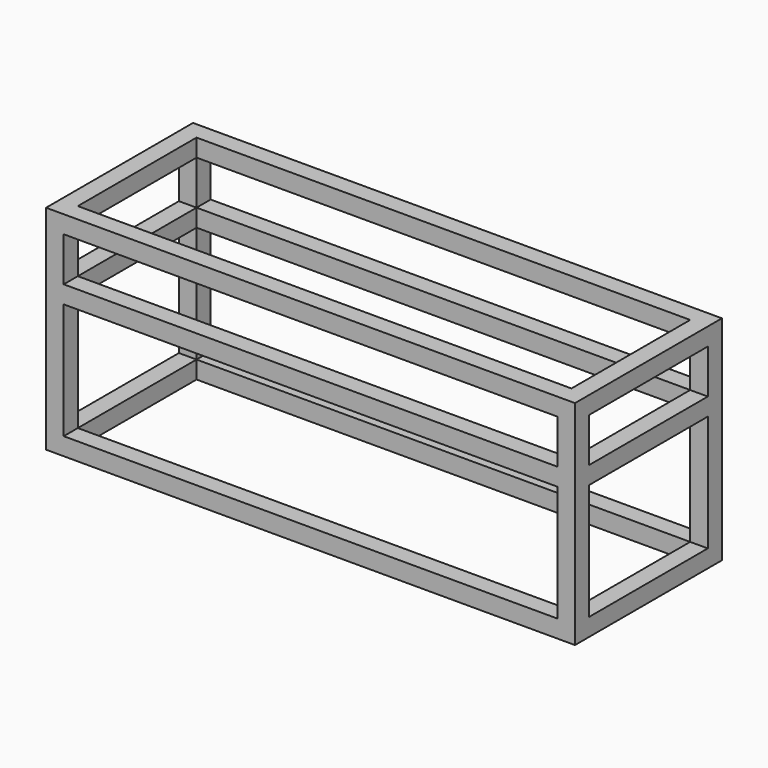
from build123d import *

# Parameters (mm, degrees)
F0_W     = 24
F0_H     = 158
F1_DEPTH = 24
F2_W     = 24
F2_H     = 24
F3_DEPTH = 202
F4_W     = 24
F4_H     = 24
F5_DEPTH = 720
F6_W     = 24
F6_H     = 24
F7_DEPTH = 280


with BuildPart() as f1:
    # F0 (on Front) → F1 (new body)
    with BuildSketch(Plane.XZ):
        Polygon((-330.027685374, 158.2459368452), (-354.027685374, 158.2459368452), (-354.027685374, 110.2459368452), (-354.027685374, 86.2459368452), (365.972314626, 86.2459368452), (365.972314626, 98.2459368452), (341.972314626, 98.2459368452), (-330.027685374, 98.2459368452), align=None)
        Polygon((365.972314626, 110.2459368452), (365.972314626, 158.2459368452), (341.972314626, 158.2459368452), (341.972314626, 98.2459368452), (365.972314626, 98.2459368452), align=None)
        Polygon((-330.027685374, 74.2459368452), (-354.027685374, 74.2459368452), (-354.027685374, 62.2459368452), (-354.027685374, -83.7540631548), (-330.027685374, -83.7540631548), align=None)
        with Locations((353.972314626, -4.7540631548)):
            Rectangle(F0_W, F0_H)
        Polygon((365.972314626, 86.2459368452), (-354.027685374, 86.2459368452), (-354.027685374, 74.2459368452), (-330.027685374, 74.2459368452), (341.972314626, 74.2459368452), (365.972314626, 74.2459368452), align=None)
        Polygon((365.972314626, 182.2459368452), (-354.027685374, 182.2459368452), (-354.027685374, 158.2459368452), (-330.027685374, 158.2459368452), (341.972314626, 158.2459368452), (365.972314626, 158.2459368452), align=None)
        Polygon((-330.027685374, -83.7540631548), (-354.027685374, -83.7540631548), (-354.027685374, -107.7540631548), (365.972314626, -107.7540631548), (365.972314626, -83.7540631548), (341.972314626, -83.7540631548), align=None)
    extrude(amount=-F1_DEPTH)

    # F2 (on face) → F3 (join)
    with BuildSketch(Plane(origin=(0, 24, 0), x_dir=(-1, 0, 0), z_dir=(0, 1, 0))):
        with Locations((-353.972314626, 86.2459368452)):
            Rectangle(F2_W, F2_H)
        with Locations((-353.972314626, -95.7540631548)):
            Rectangle(F2_W, F2_H)
        with Locations((342.027685374, 170.2459368452)):
            Rectangle(F2_W, F2_H)
        with Locations((342.027685374, -95.7540631548)):
            Rectangle(F2_W, F2_H)
        with Locations((342.027685374, 86.2459368452)):
            Rectangle(F2_W, F2_H)
        with Locations((-353.972314626, 170.2459368452)):
            Rectangle(F2_W, F2_H)
    extrude(amount=F3_DEPTH)

    # F4 (on face) → F5 (join)
    with BuildSketch(Plane.YZ.offset(365.972314626)):
        with Locations((238, 86.2459368452)):
            Rectangle(F4_W, F4_H)
        with Locations((238, 170.2459368452)):
            Rectangle(F4_W, F4_H)
        with Locations((238, -95.7540631548)):
            Rectangle(F4_W, F4_H)
    extrude(amount=-F5_DEPTH)

    # F6 (on face) → F7 (join)
    with BuildSketch(Plane.XY.offset(182.2459368452)):
        with Locations((-342.027685374, 238)):
            Rectangle(F6_W, F6_H)
        with Locations((353.972314626, 238)):
            Rectangle(F6_W, F6_H)
    extrude(amount=-F7_DEPTH)


solid = f1.part
